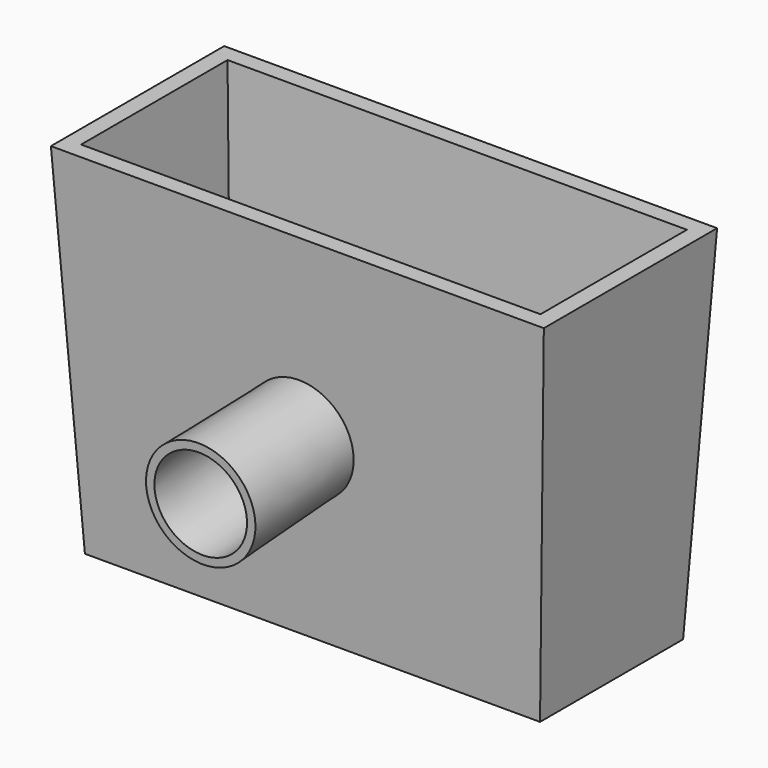
from build123d import *

# Parameters (mm, degrees)
F0_W          = 137.9242166877
F0_H          = 54.1928205639
F1_DEPTH      = 109.22
F1_TAPER      = -3
F2_T          = -5.08
F3_R          = 15.9007904293
F4_DEPTH      = 38.1
F4_TAPER      = -1
F5_T          = 2.54
F5_T3_DEPTH   = 109.5056366308
F5_T5_DEPTH   = 133.3627366899
F5_T7_DEPTH   = 109.5056366308
F5_T9_DEPTH   = 49.6313405661
F5_T11_DEPTH  = 109.5056366308
F5_T13_DEPTH  = 109.5056366308
F6_R          = 10.3601813923
F7_DEPTH      = 28.194
F7_DEPTH_BACK = 25.4


# Not quite as in the source:
# - a shell that OpenCascade refuses in one call is made with other operations: the cavity is built on its own and cut out


with BuildPart() as f1:
    # F0 (on Top) → F1 (new body)
    with BuildSketch(Plane.XY):
        with Locations((1.1629350483, -2.7910461649)):
            Rectangle(F0_W, F0_H)
    extrude(amount=F1_DEPTH, taper=F1_TAPER)

    # F2
    f2_openings = [f1.faces().sort_by_distance(p)[0] for p in [
        (1.162935, -2.791046, 109.22),
    ]]
    offset(amount=F2_T, openings=f2_openings)

    # F3 (on face) → F4 (join)
    with BuildSketch(Plane(origin=(0, -29.8055931401, -1.5620449467), x_dir=(1, 0, 0), z_dir=(0, -0.9986295348, -0.0523359562))):
        with Locations((0, 55.6432977319)):
            Circle(F3_R)
    extrude(amount=F4_DEPTH, taper=F4_TAPER)

    # F5: shell of thickness 2.54, made by hand


with BuildPart() as f5_core1:
    # F5_t2: copy of F1
    add(f1.part)

    # the walls: a layer under each face that stays
    f5_faces = [f5_core1.faces().sort_by_distance(p)[0] for p in [
        (1.1629350483, 27.1673529437, 54.61),
        (1.1629350483, -2.7910461649, 0),
        (-70.6611621221, -2.7910461649, 54.61),
        (72.0872036906, 9.6217245219, 109.22),
        (72.9870322188, -2.7910461649, 54.61),
        (-45.4478013646, -30.8414527224, 18.2033333333),
        (1.1629350483, -27.7955895152, 57.15),
        (68.0331764605, -2.7910461649, 57.15),
        (1.1629350483, 22.2134971854, 57.15),
        (-65.7073063639, -2.7910461649, 57.15),
        (-16.2333094162, -51.7416309725, 53.0079956131),
        (1.1629350483, -2.7910461649, 5.08),
    ]]
    thicken(f5_faces, amount=-F5_T, mode=Mode.SUBTRACT)

    # F5_s4 → F5_t3 (cut)
    with BuildSketch(Plane(origin=(-0.3725269372, -0.3725269372, 7.1082374087), x_dir=(0.7071067812, -0.7071067812, 0), z_dir=(-0.0522644277, -0.0522644277, 0.9972646886))):
        Polygon((-26.8076320701, -61.6755807303), (-25.0140422716, -63.5100601973), (-26.8076320701, -65.2987439692), (-28.6012218685, -63.5100601973), align=None)
    extrude(amount=F5_T3_DEPTH, mode=Mode.SUBTRACT)

    # F5_s6 → F5_t5 (cut)
    with BuildSketch(Plane.YZ.offset(-65.5184332966)):
        Polygon((-25.0413512578, 5.1067293333), (-27.6032354663, 4.9470666711), (-27.4770864474, 2.54), (-25.066716448, 2.54), align=None)
        Polygon((19.4592589279, 5.1067293333), (22.0211431364, 4.9470666711), (21.8949941176, 2.54), (19.4846241181, 2.54), align=None)
    extrude(amount=F5_T5_DEPTH, mode=Mode.SUBTRACT)

    # F5_s8 → F5_t7 (cut)
    with BuildSketch(Plane(origin=(0.3788802151, -0.3788802151, 7.229465173), x_dir=(0.7071067812, 0.7071067812, 0), z_dir=(0.0522644277, -0.0522644277, 0.9972646886))):
        Polygon((28.4522705876, -63.3157206494), (26.6586807892, -65.1502001164), (28.4522705876, -66.9388838882), (30.245860386, -65.1502001164), align=None)
    extrude(amount=F5_T7_DEPTH, mode=Mode.SUBTRACT)

    # F5_s10 → F5_t9 (cut)
    with BuildSketch(Plane.XZ.offset(-22.0246241181)):
        Polygon((65.2789382031, 5.1067293333), (67.8408224115, 4.9470666711), (67.7146733927, 2.54), (65.3043033933, 2.54), align=None)
        Polygon((-62.9530681064, 5.1067293333), (-65.5149523149, 4.9470666711), (-65.388803296, 2.54), (-62.9784332966, 2.54), align=None)
    extrude(amount=F5_T9_DEPTH, mode=Mode.SUBTRACT)

    # F5_s12 → F5_t11 (cut)
    with BuildSketch(Plane(origin=(6.0868817641, 6.0868817641, 116.1446229433), x_dir=(0.7071067812, -0.7071067812, 0), z_dir=(-0.0522644277, -0.0522644277, -0.9972646886))):
        Polygon((32.3994059273, -59.3793819539), (34.1929957257, -61.2138614209), (32.3994059273, -63.0025451928), (30.6058161288, -61.2138614209), align=None)
    extrude(amount=F5_T11_DEPTH, mode=Mode.SUBTRACT)

    # F5_s14 → F5_t13 (cut)
    with BuildSketch(Plane(origin=(-0.357279059, 0.357279059, 6.8172905608), x_dir=(-0.7071067812, -0.7071067812, 0), z_dir=(-0.0522644277, 0.0522644277, 0.9972646886))):
        Polygon((30.7547674097, -57.7392420349), (28.9611776113, -59.5737215018), (30.7547674097, -61.3624052737), (32.5483572082, -59.5737215018), align=None)
    extrude(amount=F5_T13_DEPTH, mode=Mode.SUBTRACT)

    # F5_s15 → F5_t16 (revolve, cut)
    with BuildSketch(Plane(origin=(0, -2.9121451953, 55.5670405262), x_dir=(1, 0, 0), z_dir=(0, 0.0523359562, -0.9986295348))):
        Polygon((15.9261865608, 29.8714534354), (15.9007904293, 27.3064967266), (13.3160676512, 27.3064967266), (13.3611772836, 29.8908258389), align=None)
    revolve(axis=Axis((0, -32.7177383354, 54.0049955795), (0, -0.9986295348, -0.0523359562)), mode=Mode.SUBTRACT)


with BuildPart() as f1_1:
    add(f1.part)

    # what is left inside the walls is the cavity
    f5_cavity = [f5_core1.part.solids().sort_by_distance(p)[0] for p in [
        (-13.557203, -45.430288, 53.338759),
    ]]
    add(f5_cavity, mode=Mode.SUBTRACT)

    # F6 (on face) → F7 (cut, two sides)
    with BuildSketch(Plane(origin=(0, -29.8055931401, -1.5620449467), x_dir=(1, 0, 0), z_dir=(0, -0.9986295348, -0.0523359562))) as f7_sk:
        with Locations((0, 55.7023957372)):
            Circle(F6_R)
    extrude(amount=-F7_DEPTH, mode=Mode.SUBTRACT)
    extrude(f7_sk.sketch, amount=F7_DEPTH_BACK, mode=Mode.SUBTRACT)


solid = f1_1.part
